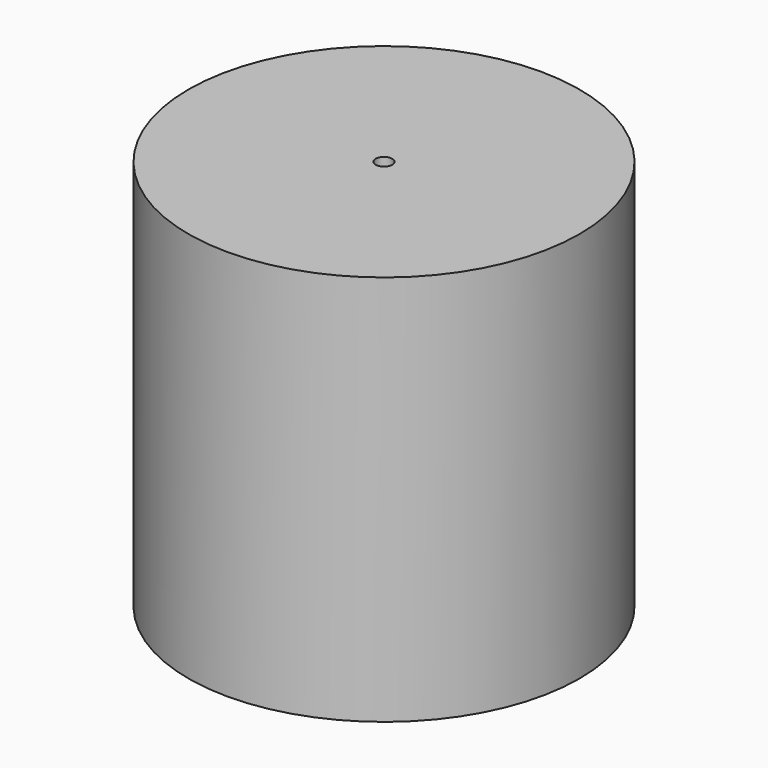
from build123d import *

# Parameters (mm, degrees)
F0_R     = 50
F1_DEPTH = 50
F3_D     = 4.2


with BuildPart() as f1:
    # F0 (on Top) → F1 (new body, symmetric)
    with BuildSketch(Plane.XY):
        Circle(F0_R)
    extrude(amount=F1_DEPTH, both=True)

    # F3 (through all)
    with Locations(Plane.XY.offset(50)):
        with Locations((0, 0)):
            Hole(F3_D / 2)


solid = f1.part
